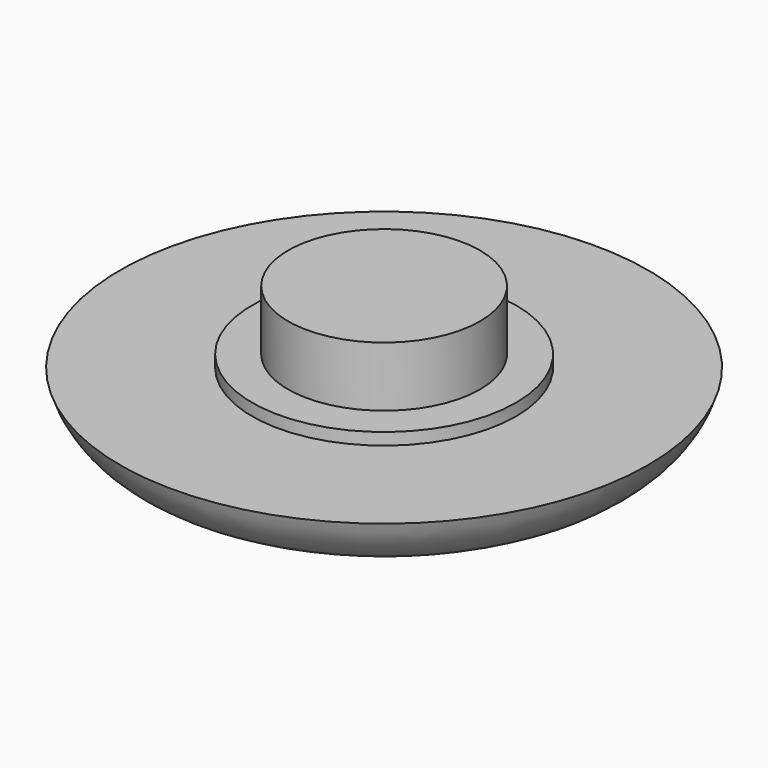
from build123d import *

# Parameters (mm, degrees)
F0_R         = 11
F0_R_2       = 5.5
F1_DEPTH     = 2.5
F0_R_3       = 4
F2_DEPTH     = 3
F3_DEPTH     = 5.5
F6_TEXT_SIZE = 5.7806594952
F7_DEPTH     = 1


# Not quite as in the source:
# - a fillet or chamfer that OpenCascade refuses, or shapes differently, is made with other operations: its cross-section is extruded or revolved along the edge and cut away or added
# - Text() gives the source's letters only with a copy of the font that has no kerning and outlines rounded to 1/6400 em; it was checked with that copy


with BuildPart() as f1:
    # F0 (on Top) → F1 (new body)
    with BuildSketch(Plane.XY):
        Circle(F0_R)
        Circle(F0_R_2, mode=Mode.SUBTRACT)
    extrude(amount=F1_DEPTH)

    # F0 (on Top) → F2 (join, through all)
    with BuildSketch(Plane.XY):
        Circle(F0_R_2)
        Circle(F0_R_3, mode=Mode.SUBTRACT)
    extrude(amount=F2_DEPTH)

    # F0 (on Top) → F3 (join, through all)
    with BuildSketch(Plane.XY):
        Circle(F0_R_3)
    extrude(amount=F3_DEPTH)

    # F4: fillet of radius 3.5 on 1 edges, made by hand

    # F4_s1 → F4_t2 (revolve, cut)
    with BuildSketch(Plane.XZ):
        with BuildLine():
            ThreePointArc((11, 2.5), (9.7375481001, 0.6937569599), (7.6458980338, 0))
            Line((7.6458980338, 0), (11, 0))
            Line((11, 0), (11, 2.5))
        make_face()
    revolve(axis=Axis((0, 0, 0), (0, 0, 1)), mode=Mode.SUBTRACT)

    # F6 (on face) → F7 (cut)
    with BuildSketch(Plane(origin=(0, 0, 0), x_dir=(1, 0, 0), z_dir=(0, 0, -1))):
        with Locations((-7.3572440497, -2.0810374183)):
            Text('JROB', F6_TEXT_SIZE, font='Open Sans', font_style=FontStyle.BOLD, text_align=(TextAlign.LEFT, TextAlign.BOTTOM))
    extrude(amount=-F7_DEPTH, mode=Mode.SUBTRACT)


solid = f1.part
